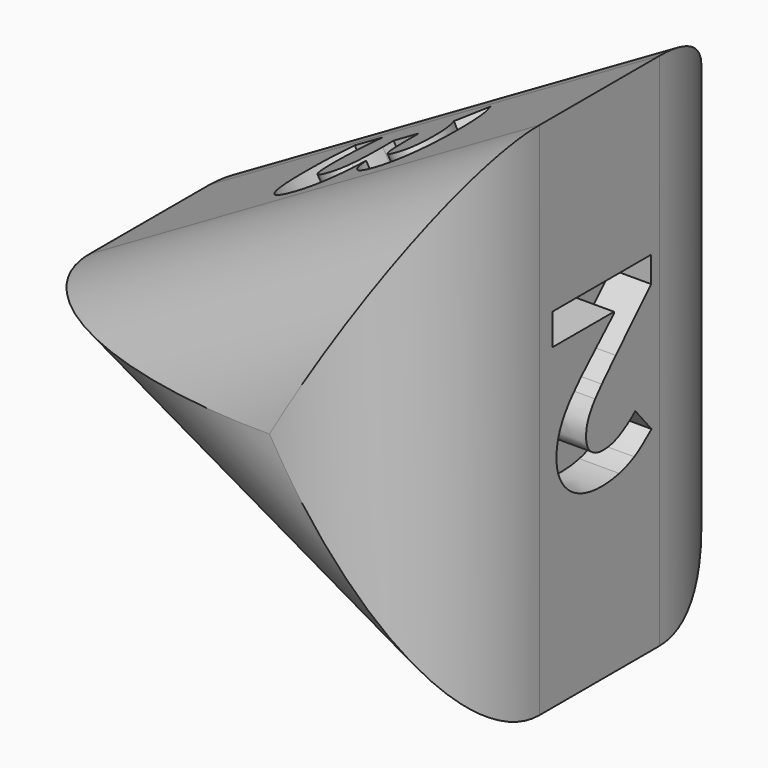
from build123d import *

# Parameters (mm, degrees)
F1_DEPTH      = 11.25
F1_DEPTH_BACK = 11.25
F2_R          = 7.49999
F3_W          = 5.6993120345
F3_H          = 2.3895553061
F6_DEPTH      = 2
F7_DEPTH      = 2
F8_DEPTH      = 2


# Not quite as in the source:
# - a fillet or chamfer is up to 0.001 mm smaller than in the source, because OpenCascade refuses the exact size


with BuildPart() as f1:
    # F0 (on Front) → F1 (new body, two sides)
    with BuildSketch(Plane.XZ) as f1_sk:
        Polygon((7.5, -12.9903810568), (7.5, 12.9903810568), (-15, 0), align=None)
    extrude(amount=F1_DEPTH)
    extrude(f1_sk.sketch, amount=-F1_DEPTH_BACK)

    # F2 (radius 7.5 in the source; OpenCascade refuses exactly that, so slightly less here)
    f2_edges = [f1.edges().sort_by_distance(p)[0] for p in [
        (7.5, 11.25, 0),
        (-3.75, 11.25, 6.495191),
        (-3.75, 11.25, -6.495191),
        (7.5, -11.25, 0),
        (-3.75, -11.25, 6.495191),
        (-3.75, -11.25, -6.495191),
    ]]
    fillet(f2_edges, radius=F2_R)

    # F3 (on face) → F6 (cut)
    with BuildSketch(Plane(origin=(-3.75, 0, -6.4951905284), x_dir=(0.8660254038, 0, -0.5), z_dir=(-0.5, 0, -0.8660254038))):
        with Locations((2.8496560172, 1.562116124)):
            Rectangle(F3_W, F3_H)
        with BuildLine():
            Line((-0.8410443106, 0.367338471), (0, 0.367338471))
            Line((0, 0.367338471), (0, 2.7568937771))
            Line((0, 2.7568937771), (-5.6028393047, 2.7568937771))
            Line((-5.6028393047, 2.7568937771), (-5.6028393047, 0.7928079458))
            Line((-5.6028393047, 0.7928079458), (-2.7037100927, -2.8484191874))
            Line((-2.7037100927, -2.8484191874), (-1.2665137854, -1.6956937498))
            Line((-1.2665137854, -1.6956937498), (-2.3103981945, -0.3970223878))
            add(Edge.make_bspline(
                [(-3.0896010117, 0.4291799644), (-2.4959226748, -0.1644983725), (-2.3103981945, -0.3970223878)],
                knots=[0, 0, 0, 1, 1, 1], degree=2))
            Line((-3.0896010117, 0.4291799644), (-1.9146126366, 0.3920750683))
            Line((-1.9146126366, 0.3920750683), (-0.8410443106, 0.367338471))
        make_face()
    extrude(amount=-F6_DEPTH, mode=Mode.SUBTRACT)

    # F4 (on face) → F7 (cut)
    with BuildSketch(Plane.YZ.offset(7.5)):
        with BuildLine():
            add(Edge.make_bspline(
                [(0.1534139825, 0), (-0.1261569639, -0.3061831776), (-0.2635343428, -0.4836289588)],
                knots=[0.5438727063, 0.5438727063, 0.5438727063, 1, 1, 1], degree=2))
            Line((0.1534139825, 0), (-1.9043553856, 0))
            add(Edge.make_bspline(
                [(-2.4683418116, -0.9662925903), (-2.2786358022, -0.49373663), (-1.9043553856, 0)],
                knots=[0, 0, 0, 0.8852247383, 0.8852247383, 0.8852247383], degree=2))
            add(Edge.make_bspline(
                [(-2.682644464, -2.110205397), (-2.682644464, -1.5001185668), (-2.4683418116, -0.9662925903)],
                knots=[0, 0, 0, 1, 1, 1], degree=2))
            add(Edge.make_bspline(
                [(-2.3322306675, -3.3525815846), (-2.682644464, -2.8091023355), (-2.682644464, -2.110205397)],
                knots=[0, 0, 0, 1, 1, 1], degree=2))
            add(Edge.make_bspline(
                [(-1.3485621865, -4.1972429397), (-1.981816871, -3.8960608337), (-2.3322306675, -3.3525815846)],
                knots=[0, 0, 0, 1, 1, 1], degree=2))
            add(Edge.make_bspline(
                [(0.1110126353, -4.4984250458), (-0.7153075019, -4.4984250458), (-1.3485621865, -4.1972429397)],
                knots=[0, 0, 0, 1, 1, 1], degree=2))
            add(Edge.make_bspline(
                [(1.2452721693, -4.3748631562), (0.7384753562, -4.4984250458), (0.1110126353, -4.4984250458)],
                knots=[0, 0, 0, 1, 1, 1], degree=2))
            add(Edge.make_bspline(
                [(2.1806742872, -4.0225187051), (1.7520689824, -4.2513012665), (1.2452721693, -4.3748631562)],
                knots=[0, 0, 0, 1, 1, 1], degree=2))
            add(Edge.make_bspline(
                [(3.2599101673, -3.2377076403), (2.609279592, -3.7937361438), (2.1806742872, -4.0225187051)],
                knots=[0, 0, 0, 1, 1, 1], degree=2))
            Line((3.2599101673, -3.2377076403), (2.2463165411, -2.036840525))
            add(Edge.make_bspline(
                [(1.2385148785, -2.7067776456), (1.72117851, -2.4712377934), (2.2463165411, -2.036840525)],
                knots=[0, 0, 0, 1, 1, 1], degree=2))
            add(Edge.make_bspline(
                [(0.2442277976, -2.9423174978), (0.755851247, -2.9423174978), (1.2385148785, -2.7067776456)],
                knots=[0, 0, 0, 1, 1, 1], degree=2))
            add(Edge.make_bspline(
                [(-0.5376872855, -2.682644464), (-0.2442277976, -2.9423174978), (0.2442277976, -2.9423174978)],
                knots=[0, 0, 0, 1, 1, 1], degree=2))
            add(Edge.make_bspline(
                [(-0.8311467735, -1.8920414356), (-0.8311467735, -2.4229714303), (-0.5376872855, -2.682644464)],
                knots=[0, 0, 0, 1, 1, 1], degree=2))
            add(Edge.make_bspline(
                [(-0.6979316112, -1.2047284243), (-0.8311467735, -1.5368010028), (-0.8311467735, -1.8920414356)],
                knots=[0, 0, 0, 1, 1, 1], degree=2))
            add(Edge.make_bspline(
                [(-0.2635343428, -0.4836289588), (-0.5647164489, -0.8726558458), (-0.6979316112, -1.2047284243)],
                knots=[0, 0, 0, 1, 1, 1], degree=2))
        make_face()
        with BuildLine():
            Line((-1.9043553856, 0), (0.1534139825, 0))
            add(Edge.make_bspline(
                [(1.0222815716, 0.9131995908), (0.4867661175, 0.3650837732), (0.1534139825, 0)],
                knots=[0, 0, 0, 0.5438727063, 0.5438727063, 0.5438727063], degree=2))
            Line((1.0222815716, 0.9131995908), (3.236742313, 3.1508281866))
            Line((3.236742313, 3.1508281866), (3.236742313, 4.4482280281))
            Line((3.236742313, 4.4482280281), (-2.9297682434, 4.4482280281))
            Line((-2.9297682434, 4.4482280281), (-2.9297682434, 2.8786058984))
            Line((-2.9297682434, 2.8786058984), (0.9141649181, 2.8786058984))
            Line((0.9141649181, 2.8786058984), (0.9141649181, 2.7955877538))
            Line((0.9141649181, 2.7955877538), (-0.2210599432, 1.7279358009))
            add(Edge.make_bspline(
                [(-1.8041966546, 0.128388526), (-1.3543541501, 0.6892436658), (-0.2210599432, 1.7279358009)],
                knots=[0, 0, 0, 1, 1, 1], degree=2))
            add(Edge.make_bspline(
                [(-1.9043553856, 0), (-1.8558274458, 0.0640162305), (-1.8041966546, 0.128388526)],
                knots=[0.8852247383, 0.8852247383, 0.8852247383, 1, 1, 1], degree=2))
        make_face()
    extrude(amount=-F7_DEPTH, mode=Mode.SUBTRACT)

    # F5 (on face) → F8 (cut)
    with BuildSketch(Plane(origin=(-3.75, 0, 6.4951905284), x_dir=(0.8660254038, 0, 0.5), z_dir=(-0.5, 0, 0.8660254038))):
        with BuildLine():
            Line((0.8145773358, 1.8911934049), (0, 1.8911934049))
            Line((0, 1.8911934049), (0, 0))
            Line((0, 0), (0, -1.5006215977))
            add(Edge.make_bspline(
                [(0.1648783041, -0.7331196022), (0.1120638425, -1.1571661487), (0, -1.5006215977)],
                knots=[0, 0, 0, 0.3899595317, 0.3899595317, 0.3899595317], degree=2))
            Line((0.1648783041, -0.7331196022), (0.2002093693, -0.7331196022))
            add(Edge.make_bspline(
                [(1.0108610311, -2.163046323), (0.422009945, -1.6536901335), (0.2002093693, -0.7331196022)],
                knots=[0, 0, 0, 1, 1, 1], degree=2))
            add(Edge.make_bspline(
                [(2.4398063334, -2.6724025124), (1.5997121172, -2.6724025124), (1.0108610311, -2.163046323)],
                knots=[0, 0, 0, 1, 1, 1], degree=2))
            add(Edge.make_bspline(
                [(4.0090944779, -1.8656765245), (3.4447788537, -2.6724025124), (2.4398063334, -2.6724025124)],
                knots=[0, 0, 0, 1, 1, 1], degree=2))
            add(Edge.make_bspline(
                [(4.5734101021, 0.3327008636), (4.5734101021, -1.0589505365), (4.0090944779, -1.8656765245)],
                knots=[0, 0, 0, 1, 1, 1], degree=2))
            add(Edge.make_bspline(
                [(3.6901334729, 3.2592907616), (4.5734101021, 2.0325176655), (4.5734101021, 0.3327008636)],
                knots=[0, 0, 0, 1, 1, 1], degree=2))
            Line((3.6901334729, 3.2592907616), (2.3848468987, 2.3819026433))
            add(Edge.make_bspline(
                [(2.8932216697, 1.3671159382), (2.7460088982, 1.8244569484), (2.3848468987, 2.3819026433)],
                knots=[0, 0, 0, 1, 1, 1], degree=2))
            add(Edge.make_bspline(
                [(3.0404344412, 0.4681366135), (3.0404344412, 0.909774928), (2.8932216697, 1.3671159382)],
                knots=[0, 0, 0, 1, 1, 1], degree=2))
            add(Edge.make_bspline(
                [(2.0217220623, -0.8077074064), (3.0404344412, -0.8077074064), (3.0404344412, 0.4681366135)],
                knots=[0, 0, 0, 1, 1, 1], degree=2))
            add(Edge.make_bspline(
                [(1.0874116723, -0.3258309343), (1.3602460089, -0.8077074064), (2.0217220623, -0.8077074064)],
                knots=[0, 0, 0, 1, 1, 1], degree=2))
            add(Edge.make_bspline(
                [(0.8145773358, 1.1983119602), (0.8145773358, 0.1560455378), (1.0874116723, -0.3258309343)],
                knots=[0, 0, 0, 1, 1, 1], degree=2))
            Line((0.8145773358, 1.1983119602), (0.8145773358, 1.8911934049))
        make_face()
        with BuildLine():
            Line((0, 0), (0, 1.8911934049))
            Line((0, 1.8911934049), (-0.6398848469, 1.8911934049))
            Line((-0.6398848469, 1.8911934049), (-0.6398848469, 1.2100889819))
            add(Edge.make_bspline(
                [(-0.9038864172, -0.4337869668), (-0.6398848469, 0.0814577336), (-0.6398848469, 1.2100889819)],
                knots=[0, 0, 0, 1, 1, 1], degree=2))
            add(Edge.make_bspline(
                [(-1.7979586496, -0.9490316671), (-1.1678879874, -0.9490316671), (-0.9038864172, -0.4337869668)],
                knots=[0, 0, 0, 1, 1, 1], degree=2))
            add(Edge.make_bspline(
                [(-2.8235409579, -0.5015048417), (-2.5045799529, -0.9490316671), (-1.7979586496, -0.9490316671)],
                knots=[0, 0, 0, 1, 1, 1], degree=2))
            add(Edge.make_bspline(
                [(-3.1425019628, 0.8862208846), (-3.1425019628, -0.0539780162), (-2.8235409579, -0.5015048417)],
                knots=[0, 0, 0, 1, 1, 1], degree=2))
            add(Edge.make_bspline(
                [(-2.9766422403, 2.1247710024), (-3.1425019628, 1.4986260141), (-3.1425019628, 0.8862208846)],
                knots=[0, 0, 0, 1, 1, 1], degree=2))
            add(Edge.make_bspline(
                [(-2.5477623659, 3.2710677833), (-2.8107825177, 2.7509159906), (-2.9766422403, 2.1247710024)],
                knots=[0, 0, 0, 1, 1, 1], degree=2))
            Line((-2.5477623659, 3.2710677833), (-4.1612143418, 3.2710677833))
            add(Edge.make_bspline(
                [(-4.6460350694, 0.6820858414), (-4.6460350694, 2.1424365349), (-4.1612143418, 3.2710677833)],
                knots=[0, 0, 0, 1, 1, 1], degree=2))
            add(Edge.make_bspline(
                [(-3.9246924889, -1.9971866004), (-4.6460350694, -1.0589505365), (-4.6460350694, 0.6820858414)],
                knots=[0, 0, 0, 1, 1, 1], degree=2))
            add(Edge.make_bspline(
                [(-1.9098403559, -2.9354226642), (-3.2033499084, -2.9354226642), (-3.9246924889, -1.9971866004)],
                knots=[0, 0, 0, 1, 1, 1], degree=2))
            add(Edge.make_bspline(
                [(-0.4956163308, -2.3779769694), (-1.0206752159, -2.9354226642), (-1.9098403559, -2.9354226642)],
                knots=[0, 0, 0, 1, 1, 1], degree=2))
            add(Edge.make_bspline(
                [(0, -1.5006215977), (-0.1753091627, -2.0379125367), (-0.4956163308, -2.3779769694)],
                knots=[0.3899595317, 0.3899595317, 0.3899595317, 1, 1, 1], degree=2))
            Line((0, -1.5006215977), (0, 0))
        make_face()
    extrude(amount=-F8_DEPTH, mode=Mode.SUBTRACT)


solid = f1.part
